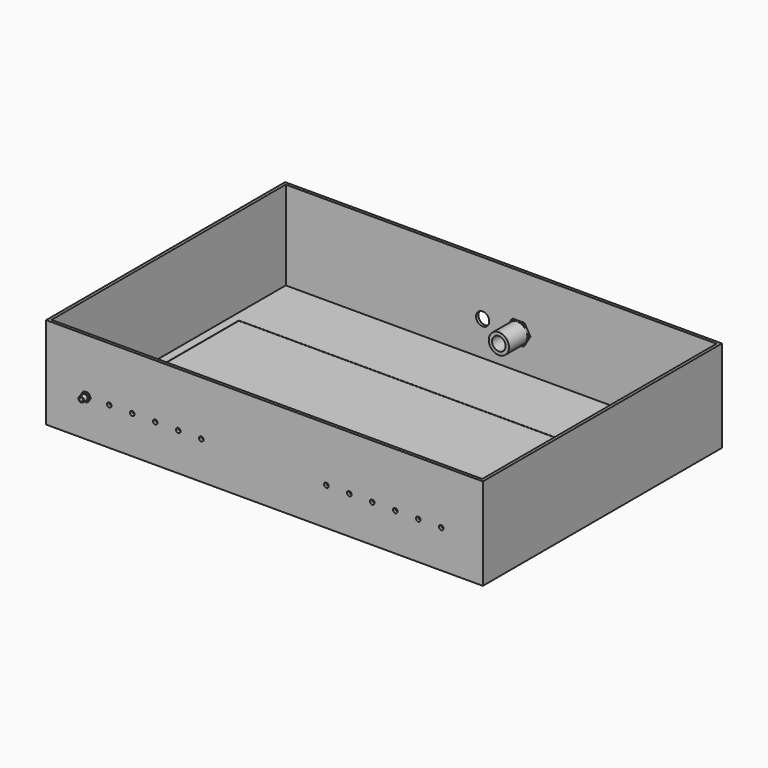
from build123d import *

# Parameters (mm, degrees)
F0_W      = 950
F0_H      = 650
F1_DEPTH  = 200
F2_T      = -2.5
F3_DEPTH  = 197.5
F4_T      = -4
F5_W      = 937
F5_H      = 637
F5_W_2    = 900
F5_H_2    = 335.756
F6_DEPTH  = 0.5
F7_R      = 5
F8_DEPTH  = 25
F9_R      = 14.3895
F10_DEPTH = 15
F11_R     = 4
F12_DEPTH = 4
F13_R     = 6
F13_R_2   = 4
F14_DEPTH = 10
F15_R     = 5
F15_R_2   = 4
F16_DEPTH = 6.5
F17_R     = 5
F17_R_2   = 4
F18_DEPTH = 4
F19_R     = 6
F19_R_2   = 5
F20_DEPTH = 150
F21_R     = 11.3895
F22_DEPTH = 4
F23_R     = 13.0309314184
F23_R_2   = 11.3895
F24_DEPTH = 25
F25_R     = 14.3895
F25_R_2   = 11.3895
F26_DEPTH = 6.5
F27_R     = 11.3895
F28_DEPTH = 4
F29_R     = 22.0019443752
F29_R_2   = 14.7554030698
F30_DEPTH = 50


# Not quite as in the source:
# - a feature names something its author has since deleted; it is built from what else it names


with BuildPart() as f1:
    # F0 (on Top) → F1 (new body)
    with BuildSketch(Plane.XY):
        Rectangle(F0_W, F0_H)
    extrude(amount=F1_DEPTH)

    # F2
    f2_openings = [f1.faces().sort_by_distance(p)[0] for p in [
        (0, 0, 200),
    ]]
    offset(amount=F2_T, openings=f2_openings)


with BuildPart() as f3:
    # F3 (new): a face of the model
    f3_faces = [f1.part.faces().sort_by_distance(p)[0] for p in [
        (0, 0, 2.5),
    ]]
    extrude(f3_faces, amount=F3_DEPTH)

    # F4
    f4_openings = [f3.faces().sort_by_distance(p)[0] for p in [
        (0, 0, 200),
    ]]
    offset(amount=F4_T, openings=f4_openings)

    # F5 (on face) → F6 (join)
    with BuildSketch(Plane.XY.offset(6.5)):
        Rectangle(F5_W, F5_H)
        Rectangle(F5_W_2, F5_H_2, mode=Mode.SUBTRACT)
    extrude(amount=F6_DEPTH)


with BuildPart() as f8_tool:
    # F7 (on face) → F8 (new body)
    with BuildSketch(Plane.XZ.offset(325)):
        with Locations((-387.5, 82.182)):
            Circle(F7_R)
        with Locations((-337.5, 82.182)):
            Circle(F7_R)
        with Locations((-287.5, 82.182)):
            Circle(F7_R)
        with Locations((-237.5, 82.182)):
            Circle(F7_R)
        with Locations((-187.5, 82.182)):
            Circle(F7_R)
        with Locations((-137.5, 82.182)):
            Circle(F7_R)
        with Locations((384.5, 82.065)):
            Circle(F7_R)
        with Locations((334.5, 82.065)):
            Circle(F7_R)
        with Locations((284.5, 82.065)):
            Circle(F7_R)
        with Locations((234.5, 82.065)):
            Circle(F7_R)
        with Locations((184.5, 82.065)):
            Circle(F7_R)
        with Locations((134.5, 82.065)):
            Circle(F7_R)
    extrude(amount=-F8_DEPTH)


with BuildPart() as f1_1:
    add(f1.part)

    # F8: cut by f8_tool
    add(f8_tool.part, mode=Mode.SUBTRACT)


with BuildPart() as f3_1:
    add(f3.part)

    # F8: cut by f8_tool
    add(f8_tool.part, mode=Mode.SUBTRACT)


with BuildPart() as f10_tool:
    # F9 (on face) → F10 (new body)
    with BuildSketch(Plane(origin=(0, 325, 0), x_dir=(-1, 0, 0), z_dir=(0, 1, 0))):
        with Locations((40.25, 82.065)):
            Circle(F9_R)
        with Locations((-38.25, 82.065)):
            Circle(F9_R)
    extrude(amount=-F10_DEPTH)


with BuildPart() as f1_2:
    add(f1_1.part)

    # F10: cut by f10_tool
    add(f10_tool.part, mode=Mode.SUBTRACT)


with BuildPart() as f3_2:
    add(f3_1.part)

    # F10: cut by f10_tool
    add(f10_tool.part, mode=Mode.SUBTRACT)


with BuildPart() as f12:
    # F11 (on face) → F12 (new body)
    with BuildSketch(Plane.XZ.offset(325)):
        Polygon((-382.5925227119, 90.682), (-392.4074772881, 90.682), (-397.3149545762, 82.182), (-392.4074772881, 73.682), (-382.5925227119, 73.682), (-377.6850454238, 82.182), align=None)
        with Locations((-387.5, 82.182)):
            Circle(F11_R, mode=Mode.SUBTRACT)
    extrude(amount=F12_DEPTH)

    # F13 (on face) → F14 (join)
    with BuildSketch(Plane.XZ.offset(329)):
        with Locations((-387.5, 82.182)):
            Circle(F13_R)
        with Locations((-387.5, 82.182)):
            Circle(F13_R_2, mode=Mode.SUBTRACT)
    extrude(amount=F14_DEPTH)

    # F15 (on face) → F16 (join)
    with BuildSketch(Plane(origin=(0, -325, 0), x_dir=(-1, 0, 0), z_dir=(0, 1, 0))):
        with Locations((387.5, 82.182)):
            Circle(F15_R)
        with Locations((387.5, 82.182)):
            Circle(F15_R_2, mode=Mode.SUBTRACT)
    extrude(amount=F16_DEPTH)

    # F17 (on face) → F18 (join)
    with BuildSketch(Plane(origin=(0, -318.5, 0), x_dir=(-1, 0, 0), z_dir=(0, 1, 0))):
        Polygon((392.4074772881, 90.682), (382.5925227119, 90.682), (377.6850454238, 82.182), (382.5925227119, 73.682), (392.4074772881, 73.682), (397.3149545762, 82.182), align=None)
        with Locations((387.5, 82.182)):
            Circle(F17_R, mode=Mode.SUBTRACT)
        with Locations((387.5, 82.182)):
            Circle(F17_R)
        with Locations((387.5, 82.182)):
            Circle(F17_R_2, mode=Mode.SUBTRACT)
    extrude(amount=F18_DEPTH)

    # F19 (on face) → F20 (join)
    with BuildSketch(Plane(origin=(0, -314.5, 0), x_dir=(-1, 0, 0), z_dir=(0, 1, 0))):
        with Locations((387.5, 82.182)):
            Circle(F19_R)
        with Locations((387.5, 82.182)):
            Circle(F19_R_2, mode=Mode.SUBTRACT)
    extrude(amount=F20_DEPTH)


with BuildPart() as f22:
    # F21 (on face) → F22 (new body)
    with BuildSketch(Plane(origin=(0, 325, 0), x_dir=(-1, 0, 0), z_dir=(0, 1, 0))):
        Polygon((-28.1578817366, 99.5450615883), (-48.3421182634, 99.5450615883), (-58.4342365269, 82.065), (-48.3421182634, 64.5849384117), (-28.1578817366, 64.5849384117), (-18.0657634731, 82.065), align=None)
        with Locations((-38.25, 82.065)):
            Circle(F21_R, mode=Mode.SUBTRACT)
    extrude(amount=F22_DEPTH)

    # F23 (on face) → F24 (join)
    with BuildSketch(Plane(origin=(0, 329, 0), x_dir=(-1, 0, 0), z_dir=(0, 1, 0))):
        with Locations((-38.25, 82.065)):
            Circle(F23_R)
        with Locations((-38.25, 82.065)):
            Circle(F23_R_2, mode=Mode.SUBTRACT)
    extrude(amount=F24_DEPTH)

    # F25 (on face) → F26 (join)
    with BuildSketch(Plane.XZ.offset(-325)):
        with Locations((38.25, 82.065)):
            Circle(F25_R)
        with Locations((38.25, 82.065)):
            Circle(F25_R_2, mode=Mode.SUBTRACT)
    extrude(amount=F26_DEPTH)

    # F27 (on face) → F28 (join)
    with BuildSketch(Plane.XZ.offset(-318.5)):
        Polygon((50.9528285077, 104.0669443752), (25.5471714923, 104.0669443752), (12.8443429845, 82.065), (25.5471714923, 60.0630556248), (50.9528285077, 60.0630556248), (63.6556570155, 82.065), align=None)
        with Locations((38.25, 82.065)):
            Circle(F27_R, mode=Mode.SUBTRACT)
    extrude(amount=F28_DEPTH)

    # F29 (on face) → F30 (join)
    with BuildSketch(Plane.XZ.offset(-314.5)):
        with Locations((38.25, 82.065)):
            Circle(F29_R)
        with Locations((38.25, 82.065)):
            Circle(F29_R_2, mode=Mode.SUBTRACT)
    extrude(amount=F30_DEPTH)


solid = Compound([f1_2.part, f3_2.part, f12.part, f22.part])
